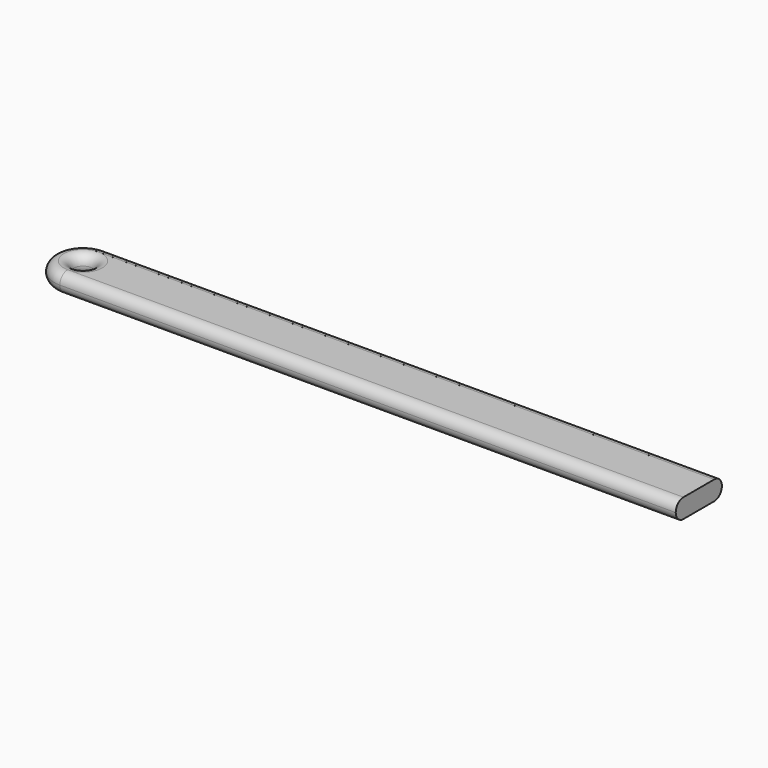
from build123d import *

# Parameters (mm, degrees)
F1_DEPTH = 3.175
F2_R     = 3.175
F3_DEPTH = 6.351
F4_R     = 3.17499
F5_R     = 3.17499


# Not quite as in the source:
# - a fillet or chamfer is up to 0.001 mm smaller than in the source, because OpenCascade refuses the exact size


with BuildPart() as f1:
    # F0 (on Top) → F1 (new body, symmetric)
    with BuildSketch(Plane.XY):
        with BuildLine():
            Line((101.6, -9.525), (101.6, 9.525))
            Line((101.6, 9.525), (-101.6, 9.525))
            ThreePointArc((-101.6, 9.525), (-111.125, 0), (-101.6, -9.525))
            Line((-101.6, -9.525), (101.6, -9.525))
        make_face()
    extrude(amount=F1_DEPTH, both=True)

    # F2 (on face) → F3 (cut, through all)
    with BuildSketch(Plane.XY.offset(3.175)):
        with Locations((-101.6, 0)):
            Circle(F2_R)
    extrude(amount=-F3_DEPTH, mode=Mode.SUBTRACT)

    # F4 (radius 3.175 in the source; OpenCascade refuses exactly that, so slightly less here)
    f4_edges = [f1.edges().sort_by_distance(p)[0] for p in [
        (0, -9.525, 3.175),
        (-104.775, 0, 3.175),
    ]]
    fillet(f4_edges, radius=F4_R)

    # F5 (radius 3.175 in the source; OpenCascade refuses exactly that, so slightly less here)
    f5_edges = [f1.edges().sort_by_distance(p)[0] for p in [
        (0, -9.525, -3.175),
        (-104.775, 0, -3.175),
    ]]
    fillet(f5_edges, radius=F5_R)


solid = f1.part
